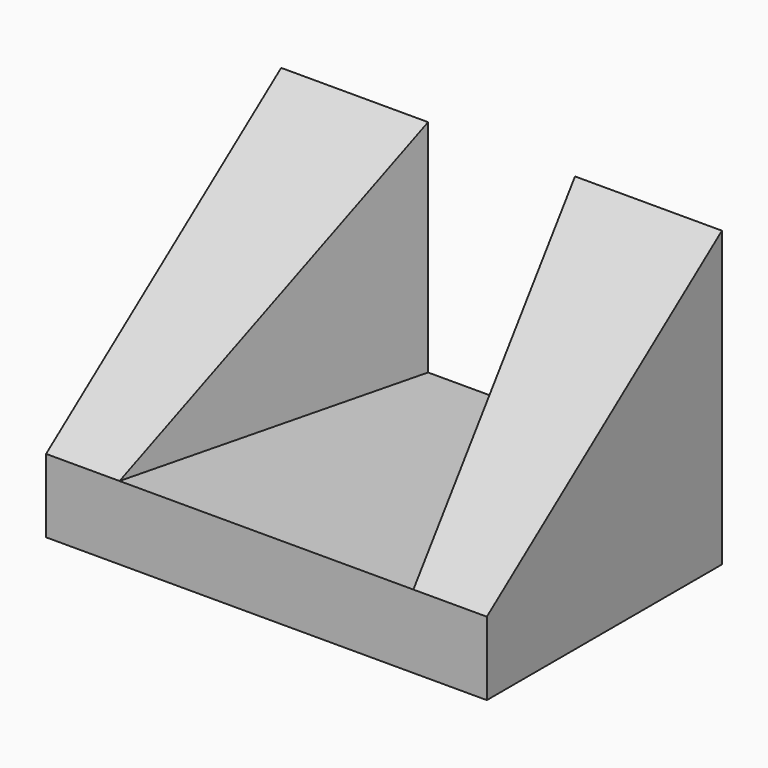
from build123d import *

# Parameters (mm, degrees)
F0_W     = 60
F0_H     = 40
F1_DEPTH = 10
F3_DEPTH = 30
F4_SIZE2 = 39.99999
F4_SIZE  = 29.99999


# Not quite as in the source:
# - a fillet or chamfer is up to 0.001 mm smaller than in the source, because OpenCascade refuses the exact size


with BuildPart() as f1:
    # F0 (on Top) → F1 (new body)
    with BuildSketch(Plane.XY):
        with Locations((30, 20)):
            Rectangle(F0_W, F0_H)
    extrude(amount=F1_DEPTH)

    # F2 (on face) → F3 (join)
    with BuildSketch(Plane.XY.offset(10)):
        Polygon((20, 40), (0, 40), (0, 0), (10, 0), align=None)
        Polygon((60, 0), (60, 40), (40, 40), (50, 0), align=None)
    extrude(amount=F3_DEPTH)

    # F4 (size 30 and 40 in the source; OpenCascade refuses exactly that, so slightly less here)
    f4_edges = [f1.edges().sort_by_distance(p)[0] for p in [
        (55, 0, 40),
        (5, 0, 40),
    ]]
    f4_side = f1.faces().sort_by_distance((0.72111, 0, 20))[0]
    chamfer(f4_edges, length=F4_SIZE, length2=F4_SIZE2, reference=f4_side)


solid = f1.part
